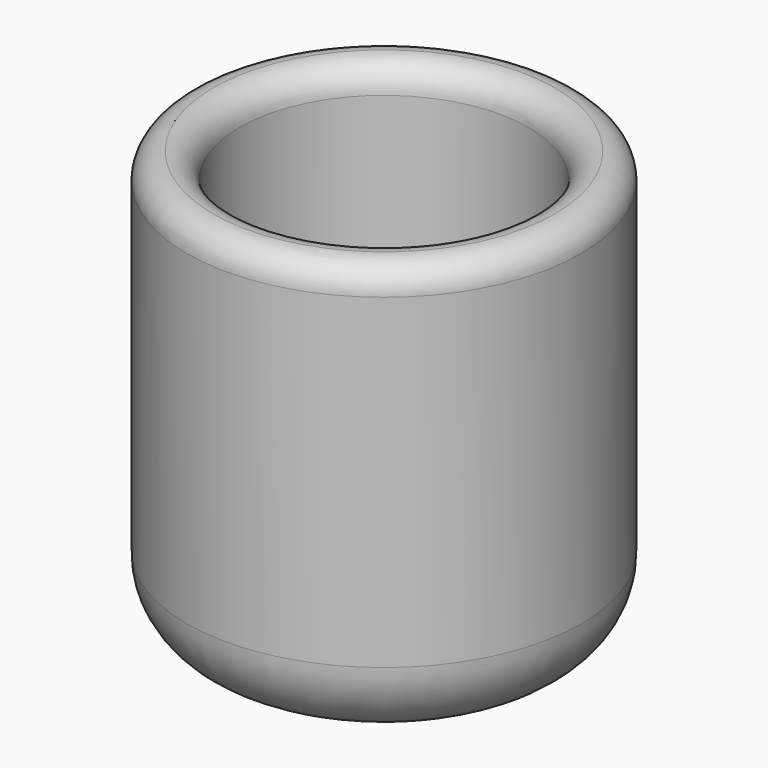
from build123d import *

# Parameters (mm, degrees)
F0_R     = 37.5
F0_R_2   = 27.5
F1_DEPTH = 82
F2_DEPTH = 5
F3_R     = 15
F4_R     = 5
F5_R     = 4.99999


# Not quite as in the source:
# - a fillet or chamfer is up to 0.001 mm smaller than in the source, because OpenCascade refuses the exact size


with BuildPart() as f1:
    # F0 (on Top) → F1 (new body)
    with BuildSketch(Plane.XY):
        Circle(F0_R)
        Circle(F0_R_2, mode=Mode.SUBTRACT)
    extrude(amount=F1_DEPTH)

    # F0 (on Top) → F2 (join)
    with BuildSketch(Plane.XY):
        Circle(F0_R_2)
    extrude(amount=F2_DEPTH)

    # F3
    f3_edges = [f1.edges().sort_by_distance(p)[0] for p in [
        (-37.5, 0, 0),
    ]]
    fillet(f3_edges, radius=F3_R)

    # F4
    f4_edges = [f1.edges().sort_by_distance(p)[0] for p in [
        (-37.5, 0, 82),
    ]]
    fillet(f4_edges, radius=F4_R)

    # F5 (radius 5 in the source; OpenCascade refuses exactly that, so slightly less here)
    f5_edges = [f1.edges().sort_by_distance(p)[0] for p in [
        (-27.5, 0, 82),
    ]]
    fillet(f5_edges, radius=F5_R)


solid = f1.part
